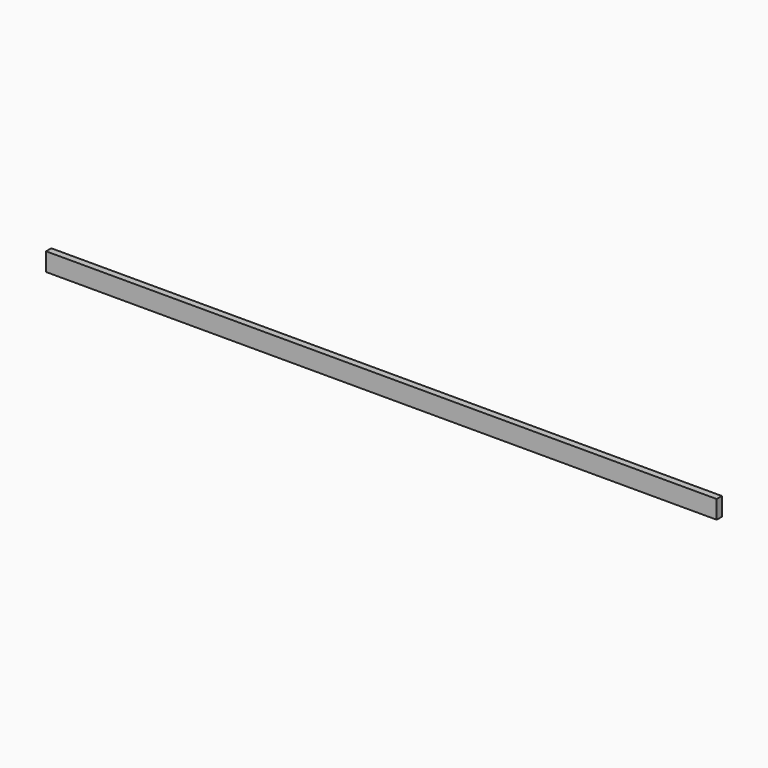
from build123d import *

# Parameters (mm, degrees)
F0_W     = 1866.9
F0_H     = 50.8
F1_DEPTH = 18.25625


# Not quite as in the source:
# - a length typed as a fraction of an inch, garbled in the dataset ("3 / 203.2 mm" for 3/8 in), is restored


with BuildPart() as f1:
    # F0 (on Front) → F1 (new body)
    with BuildSketch(Plane.XZ):
        with Locations((822.3223254204, 12.7396940529)):
            Rectangle(F0_W, F0_H)
    extrude(amount=F1_DEPTH)


solid = f1.part
